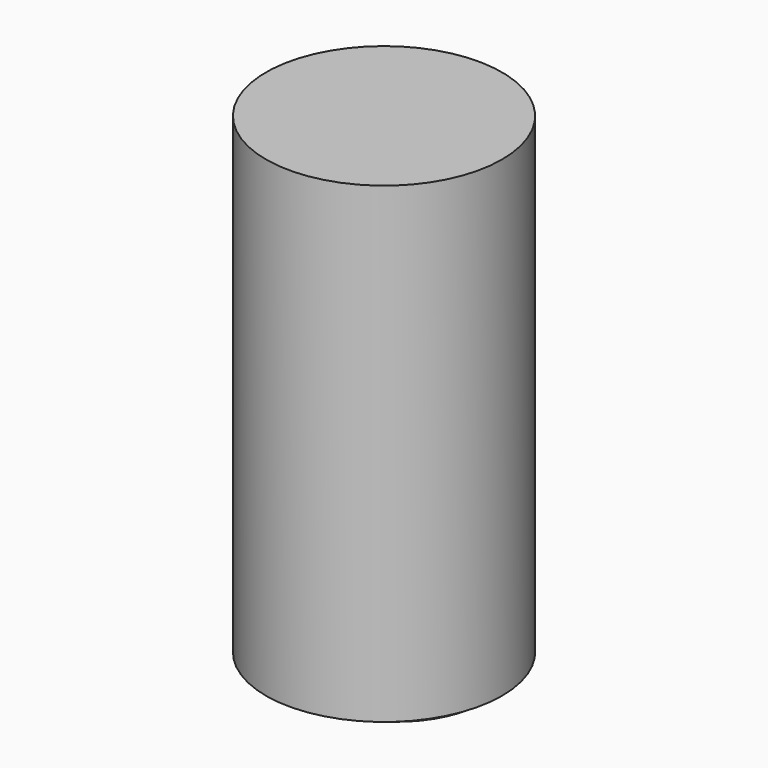
from build123d import *

# Parameters (mm, degrees)
F1_DEPTH               = 1.5
DRAFT_F1_DRAFTED_ANGLE = 3
F0_R                   = 7.5
F2_DEPTH               = 30


# Not quite as in the source:
# - an extrude with a draft is written as a straight extrude whose walls are then drafted


with BuildPart() as f1:
    # F0 (on Top) → F1 (new body)
    with BuildSketch(Plane.XY):
        with BuildLine():
            ThreePointArc((0, -4.5), (5.5360295397, 1.15), (0, 6.8))
            Line((0, 6.8), (-3.1708920755, 0))
            Line((-3.1708920755, 0), (-5.6290794164, 0))
            ThreePointArc((-5.6290794164, 0), (-6.0533434851, -0.1757359313), (-6.2290794164, -0.6))
            ThreePointArc((-6.2290794164, -0.6), (-6.0533434851, -1.0242640687), (-5.6290794164, -1.2))
            Line((-5.6290794164, -1.2), (-3.7304612652, -1.2))
            Line((-3.7304612652, -1.2), (-5.2692765372, -4.5))
            Line((-5.2692765372, -4.5), (-4.0692765372, -4.5))
            Line((-4.0692765372, -4.5), (-2.5304612652, -1.2))
            Line((-2.5304612652, -1.2), (0, -1.2))
            Line((0, -1.2), (0, -4.5))
        make_face()
        Polygon((0, 0), (-1.9708920755, 0), (0, 4.2265916954), align=None, mode=Mode.SUBTRACT)
        with BuildLine():
            Line((1.2, -3.1024510274), (1.2, 5.4024510274))
            ThreePointArc((1.2, 5.4024510274), (4.3360295397, 1.15), (1.2, -3.1024510274))
        make_face(mode=Mode.SUBTRACT)
    extrude(amount=-F1_DEPTH)

    # draft_F1_drafted
    draft_f1_drafted_walls = [f1.faces().sort_by_distance(p)[0] for p in [
        (5.5360295397, 1.15, -1),
        (1.2, 1.15, -1),
        (4.3360295397, 1.15, -1),
        (-0.9854460377, 2.1132958477, -1),
        (-0.9854460377, 0, -1),
        (0, 2.1132958477, -1),
        (-1.2652306326, -1.2, -1),
        (-3.2998689012, -2.85, -1),
        (-4.6692765372, -4.5, -1),
        (-4.4998689012, -2.85, -1),
        (-4.6797703408, -1.2, -1),
        (-6.2290794164, -0.6, -1),
        (-4.3999857459, 0, -1),
        (-1.5854460377, 3.4, -1),
        (0, -2.85, -1),
    ]]
    draft(draft_f1_drafted_walls, neutral_plane=Plane(origin=(0, 0, 0), x_dir=(1, 0, 0), z_dir=(0, 0, -1)), angle=DRAFT_F1_DRAFTED_ANGLE)


with BuildPart() as f2:
    # F0 (on Top) → F2 (new body)
    with BuildSketch(Plane.XY):
        Circle(F0_R)
        with BuildLine():
            Line((-3.1708920755, 0), (0, 6.8))
            ThreePointArc((0, 6.8), (5.5360295397, 1.15), (0, -4.5))
            Line((0, -4.5), (0, -1.2))
            Line((0, -1.2), (-2.5304612652, -1.2))
            Line((-2.5304612652, -1.2), (-4.0692765372, -4.5))
            Line((-4.0692765372, -4.5), (-5.2692765372, -4.5))
            Line((-5.2692765372, -4.5), (-3.7304612652, -1.2))
            Line((-3.7304612652, -1.2), (-5.6290794164, -1.2))
            ThreePointArc((-5.6290794164, -1.2), (-6.0533434851, -1.0242640687), (-6.2290794164, -0.6))
            ThreePointArc((-6.2290794164, -0.6), (-6.0533434851, -0.1757359313), (-5.6290794164, 0))
            Line((-5.6290794164, 0), (-3.1708920755, 0))
        make_face(mode=Mode.SUBTRACT)
        with BuildLine():
            ThreePointArc((0, -4.5), (5.5360295397, 1.15), (0, 6.8))
            Line((0, 6.8), (-3.1708920755, 0))
            Line((-3.1708920755, 0), (-5.6290794164, 0))
            ThreePointArc((-5.6290794164, 0), (-6.0533434851, -0.1757359313), (-6.2290794164, -0.6))
            ThreePointArc((-6.2290794164, -0.6), (-6.0533434851, -1.0242640687), (-5.6290794164, -1.2))
            Line((-5.6290794164, -1.2), (-3.7304612652, -1.2))
            Line((-3.7304612652, -1.2), (-5.2692765372, -4.5))
            Line((-5.2692765372, -4.5), (-4.0692765372, -4.5))
            Line((-4.0692765372, -4.5), (-2.5304612652, -1.2))
            Line((-2.5304612652, -1.2), (0, -1.2))
            Line((0, -1.2), (0, -4.5))
        make_face()
        Polygon((0, 0), (-1.9708920755, 0), (0, 4.2265916954), align=None, mode=Mode.SUBTRACT)
        with BuildLine():
            Line((1.2, -3.1024510274), (1.2, 5.4024510274))
            ThreePointArc((1.2, 5.4024510274), (4.3360295397, 1.15), (1.2, -3.1024510274))
        make_face(mode=Mode.SUBTRACT)
        Polygon((0, 4.2265916954), (-1.9708920755, 0), (0, 0), align=None)
        with BuildLine():
            ThreePointArc((1.2, -3.1024510274), (4.3360295397, 1.15), (1.2, 5.4024510274))
            Line((1.2, 5.4024510274), (1.2, -3.1024510274))
        make_face()
    extrude(amount=F2_DEPTH)


solid = Compound([f1.part, f2.part])
